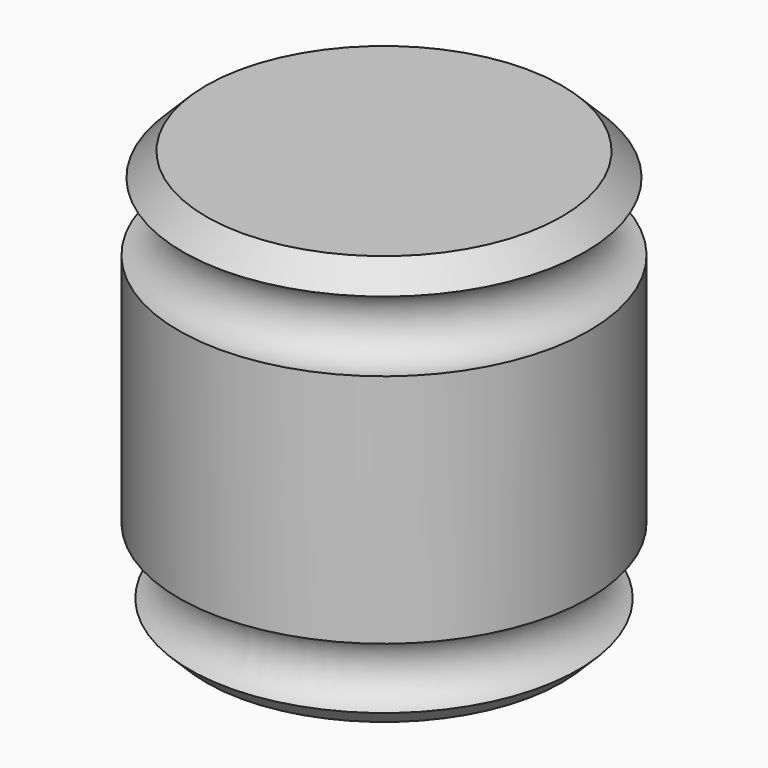
from build123d import *


# Not quite as in the source:
# - a fillet or chamfer that OpenCascade refuses, or shapes differently, is made with other operations: its cross-section is extruded or revolved along the edge and cut away or added


with BuildPart() as f2:
    # F0 (on Front) → F2 (revolve)
    with BuildSketch(Plane.XZ):
        with BuildLine():
            Line((-30.0974734128, 0), (8.0025265872, 0))
            Line((8.0025265872, 0), (8.0025265872, 76.2))
            Line((8.0025265872, 76.2), (-30.0974734128, 76.2))
            Line((-30.0974734128, 76.2), (-30.0974734128, 71.8881083488))
            ThreePointArc((-30.0974734128, 71.8881083488), (-23.7474734128, 65.5381083488), (-30.0974734128, 59.1881083488))
            Line((-30.0974734128, 59.1881083488), (-30.0974734128, 15.4437847272))
            ThreePointArc((-30.0974734128, 15.4437847272), (-23.7474734128, 9.0937847272), (-30.0974734128, 2.7437847272))
            Line((-30.0974734128, 2.7437847272), (-30.0974734128, 0))
        make_face()
    revolve(axis=Axis((8.0025265872, 0, 38.1), (0, 0, 1)))

    # F3: chamfer of 5.08 on 2 edges, made by hand

    # F3_s1 → F3_t2 (revolve, cut)
    with BuildSketch(Plane.XZ):
        Polygon((-25.0174734128, 76.2), (-30.0974734128, 71.12), (-30.0974734128, 76.2), align=None)
    revolve(axis=Axis((8.0025265872, 0, 76.2), (0, 0, 1)), mode=Mode.SUBTRACT)

    # F3_s3 → F3_t4 (revolve, cut)
    with BuildSketch(Plane.XZ):
        Polygon((-30.0974734128, 5.08), (-25.0174734128, 0), (-30.0974734128, 0), align=None)
    revolve(axis=Axis((8.0025265872, 0, 0), (0, 0, 1)), mode=Mode.SUBTRACT)


solid = f2.part
